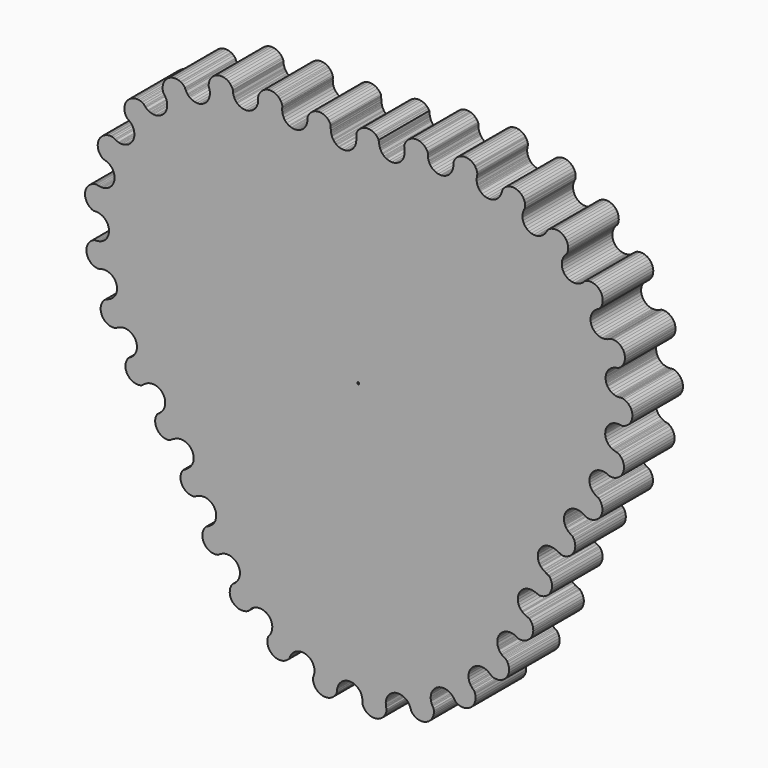
from build123d import *

# Parameters (mm, degrees)
F0_R     = 0.1932686
F1_DEPTH = 12.7


# Not quite as in the source:
# - ends of sketch curves that miss each other by under 0.0002 mm in the source are joined


with BuildPart() as f1:
    # F0 (on Front) → F1 (new body)
    with BuildSketch(Plane.XZ):
        Polygon((-7.2596502, -52.0065254), (-7.258685, -52.006754), (-6.7694048, -52.0724638), (-6.322441, -52.044346), (-6.2991238, -52.0413742), (-6.255639, -52.0358624), (-5.9557158, -51.9563604), (-5.7304432, -51.8810748), (-5.6054752, -51.8198608), (-5.2589684, -51.6220202), (-4.8862488, -51.2983226), (-4.5838364, -50.9081278), (-4.445508, -50.6309884), (-4.3810682, -50.4785376), (-4.38277, -50.2927112), (-4.3556936, -50.1496838), (-4.3439588, -49.9317772), (-4.2878502, -49.7120926), (-4.283329, -49.6734592), (-4.2580052, -49.5952272), (-4.2380408, -49.5170968), (-4.2218102, -49.4535968), (-4.1919906, -49.3912906), (-4.1470072, -49.2522764), (-4.1313354, -49.2039148), (-3.8906704, -48.7730292), (-3.5705796, -48.3973886), (-3.1833566, -48.0913948), (-2.7438604, -47.8668334), (-2.5818084, -47.8209356), (-2.5621996, -47.8124266), (-2.5180036, -47.8028508), (-2.2690074, -47.7323404), (-2.1470366, -47.7225868), (-2.0798282, -47.708058), (-1.9344386, -47.7056196), (-1.8059654, -47.695358), (-1.7770348, -47.6930466), (-1.7760188, -47.693072), (-1.7021048, -47.7017334), (-1.6081248, -47.7001586), (-1.586357, -47.699803), (-1.585341, -47.6998792), (-1.3438886, -47.7437196), (-1.2858496, -47.7505268), (-1.2595606, -47.7590358), (-1.0997692, -47.7880426), (-0.6406896, -47.9692462), (-0.225806, -48.2365558), (0.1289812, -48.5796336), (0.4100068, -48.9853478), (0.6064758, -49.4381028), (0.6447536, -49.614963), (0.6720078, -49.6904772), (0.697357, -49.8581172), (0.7108444, -49.9204742), (0.7113524, -49.9506748), (0.7457948, -50.178462), (0.735965, -50.3910092), (0.7487158, -50.5372878), (0.744474, -50.5759974), (0.7261352, -50.7430532), (0.7559802, -50.8404876), (0.782955, -50.9285748), (0.8832596, -51.1949192), (1.1438382, -51.613816), (1.4810994, -51.9738102), (1.8554192, -52.2419326), (1.8963132, -52.267485), (2.2015704, -52.4057372), (2.3973028, -52.4799306), (2.5652476, -52.5190466), (2.6849324, -52.5390872), (2.931795, -52.5804384), (2.9387546, -52.580667), (2.9445458, -52.5808448), (3.4289492, -52.5660874), (3.4299398, -52.5659604), (3.9106348, -52.4550386), (4.360418, -52.2524736), (4.7620682, -51.9660632), (5.1001168, -51.6067802), (5.361559, -51.1884422), (5.5226712, -50.7633732), (5.5394352, -50.7090426), (5.5643018, -50.5604018), (5.5986172, -50.227865), (5.5079392, -49.938178), (5.489067, -49.762537), (5.4499256, -49.6022376), (5.4286404, -49.1090712), (5.4507638, -48.9657898), (5.4527196, -48.8699302), (5.4956456, -48.675036), (5.5039514, -48.6212642), (5.5129176, -48.5967024), (5.558917, -48.387889), (5.7570878, -47.9358198), (6.0396882, -47.5310962), (6.3957708, -47.189263), (6.8117212, -46.9235028), (7.2715374, -46.7439756), (7.2725026, -46.7436962), (7.7585062, -46.6573362), (8.2520028, -46.6674454), (8.734044, -46.7736174), (8.869172, -46.8328756), (8.9234772, -46.8484966), (9.0284554, -46.9027002), (9.1861386, -46.9718136), (9.2536264, -47.0189306), (9.3620844, -47.0749376), (9.5617284, -47.2340686), (9.5908368, -47.2543886), (9.602597, -47.2666314), (9.7480882, -47.3825824), (10.066655, -47.7596454), (10.1220524, -47.8597976), (10.2047802, -48.009429), (10.20953, -48.0158044), (10.2166674, -48.0309174), (10.3055166, -48.1915724), (10.3282242, -48.2627686), (10.3321104, -48.274859), (10.4206294, -48.4619808), (10.4852216, -48.719613), (10.5323132, -48.8379516), (10.550398, -48.9359956), (10.576814, -48.9758482), (10.8056426, -49.2775748), (11.1644684, -49.5958368), (11.1806228, -49.6084098), (11.452225, -49.7672614), (11.6798852, -49.8815106), (11.7551454, -49.9075202), (12.179046, -50.0242586), (12.6711964, -50.0599202), (13.160883, -49.9989094), (13.6292336, -49.8435122), (13.6301734, -49.8431058), (14.0592048, -49.599342), (14.4324578, -49.2765334), (14.735556, -48.8871514), (14.9568662, -48.4460804), (15.087854, -47.9703384), (15.1098504, -47.6671132), (15.1120094, -47.3911168), (15.0335996, -46.9799924), (14.8506688, -46.710219), (14.7757388, -46.5326476), (14.692884, -46.391068), (14.5313908, -45.9244446), (14.5081244, -45.7555346), (14.4884648, -45.6837034), (14.4779746, -45.536485), (14.4640554, -45.435266), (14.4671034, -45.3838056), (14.4534128, -45.191172), (14.5151094, -44.7012568), (14.6711924, -44.2328046), (14.9156928, -43.8037986), (15.2391872, -43.4307234), (15.6292296, -43.12793), (15.6300932, -43.1273966), (16.071723, -42.9065182), (16.547973, -42.7760384), (17.0405044, -42.7409864), (17.5304196, -42.802683), (17.6652174, -42.8476156), (17.7405538, -42.8621444), (17.88287, -42.9201326), (17.9988718, -42.9587914), (18.051907, -42.9890174), (18.19783, -43.0484788), (18.6099704, -43.3204366), (18.9611508, -43.6675784), (19.0228982, -43.758866), (19.1610488, -43.9143902), (19.3112644, -44.1708032), (19.3882518, -44.2696346), (19.4080384, -44.30903), (19.4484752, -44.34332), (19.7320408, -44.553251), (20.1783696, -44.763817), (20.3202032, -44.7992246), (20.5983078, -44.8686174), (20.6884778, -44.8847972), (20.9026252, -44.8951096), (20.9478372, -44.897294), (21.0921346, -44.894627), (21.2536024, -44.8916044), (21.2793072, -44.887769), (21.2991446, -44.8847972), (21.7514932, -44.7860166), (22.2038164, -44.588684), (22.6089464, -44.3069218), (22.6097338, -44.3062614), (22.9521004, -43.9508646), (23.2185718, -43.535473), (23.3988864, -43.076114), (23.48611, -42.5903898), (23.4769152, -42.0969694), (23.391495, -41.7058348), (23.3520996, -41.5700972), (23.3222546, -41.501695), (23.2649776, -41.391332), (23.1707944, -41.2099252), (22.9620826, -41.0350716), (22.8696266, -40.9200858), (22.7466652, -40.8055318), (22.584029, -40.5798782), (22.5667062, -40.5613362), (22.542373, -40.5220932), (22.4582228, -40.4053294), (22.4253806, -40.3333458), (22.306788, -40.142033), (22.133687, -39.6800832), (22.0540072, -39.1932414), (22.0708474, -38.700202), (22.1835726, -38.2199134), (22.3877886, -37.7708668), (22.675723, -37.3702834), (22.6763834, -37.3695214), (22.7885498, -37.2647464), (22.8252782, -37.2204234), (22.8260148, -37.2197122), (22.9089712, -37.1522752), (23.036911, -37.0327936), (23.1173528, -36.9829588), (23.2088436, -36.9085876), (23.4017058, -36.8066828), (23.4562142, -36.7729008), (23.4886754, -36.7607342), (23.6450124, -36.678108), (24.1177826, -36.5371634), (24.6089424, -36.491164), (25.0996704, -36.5418624), (25.5710436, -36.6873282), (25.7974846, -36.8097562), (25.8438904, -36.8276124), (25.9229098, -36.8775488), (26.0050026, -36.921948), (26.0180328, -36.932743), (26.0432296, -36.9536218), (26.2608822, -37.0912136), (26.390219, -37.214175), (26.4523982, -37.2732808), (26.5811, -37.3673624), (26.6543282, -37.4470422), (26.6817094, -37.4768364), (26.901267, -37.5745756), (27.0568674, -37.6342656), (27.543125, -37.7176538), (28.0362914, -37.7045728), (28.5174436, -37.5955306), (28.895929, -37.4268746), (28.9921188, -37.3777256), (29.1585904, -37.2599712), (29.2089078, -37.2243858), (29.4217852, -37.0561616), (29.4921432, -36.9819682), (29.7636184, -36.6633506), (29.7642026, -36.6625378), (30.0047406, -36.2318046), (30.156658, -35.7624126), (30.214062, -35.2723958), (30.1747682, -34.780601), (30.0403006, -34.3059512), (29.8845478, -34.0011512), (29.7804078, -33.8218272), (29.7726862, -33.8120736), (29.5570402, -33.5674208), (29.3539164, -33.471612), (29.215334, -33.3690722), (29.0514024, -33.2800706), (28.8873946, -33.1436726), (28.8390838, -33.1138276), (28.7354772, -33.017333), (28.6718502, -32.9644248), (28.6509714, -32.9386438), (28.477845, -32.7774046), (28.1891486, -32.3769482), (28.1318208, -32.2513452), (28.1035252, -32.2071238), (28.0550874, -32.083248), (27.9841198, -31.9278508), (27.9686258, -31.8622426), (27.9237186, -31.7473584), (27.8370538, -31.2613802), (27.8468582, -30.7678074), (27.9527762, -30.2856392), (28.1507184, -29.8334176), (28.1512264, -29.8325286), (28.4335982, -29.4276018), (28.7895284, -29.08554), (29.2053772, -28.8195004), (29.6651172, -28.6396684), (29.815282, -28.6128968), (29.8533566, -28.6003746), (29.9557948, -28.5878524), (30.1511208, -28.553029), (30.2282098, -28.554553), (30.3433988, -28.5404814), (30.6410868, -28.5627572), (30.6446936, -28.5628334), (30.6460652, -28.5631382), (30.8356762, -28.5773368), (31.0711088, -28.6427672), (31.090997, -28.645358), (31.1406286, -28.6620966), (31.3113166, -28.7095184), (31.3718956, -28.7401), (31.5587634, -28.8031428), (31.6428882, -28.8515044), (31.7260478, -28.8993072), (31.8625982, -28.953714), (32.0957448, -29.1049202), (32.3817742, -29.16301), (32.6060816, -29.1638736), (32.9381358, -29.1463476), (33.4161892, -29.0247324), (33.8613496, -28.8121852), (34.256472, -28.5168594), (34.586418, -28.1501342), (34.8384622, -27.7261066), (34.8388686, -27.7251922), (35.003359, -27.2601182), (35.0609154, -26.862024), (35.071939, -26.7342874), (35.0595438, -26.4992358), (35.025457, -26.1909814), (35.0120204, -26.1382002), (34.8748604, -25.7047492), (34.6371418, -25.2725174), (34.3196672, -24.8949718), (34.2319864, -24.8247408), (34.0772242, -24.7827546), (33.8386166, -24.6641366), (33.6741516, -24.6085868), (33.4651858, -24.4883686), (33.3699104, -24.449659), (32.9583542, -24.1785902), (32.8722482, -24.0936272), (32.768413, -24.015954), (32.4390004, -23.6494828), (32.1874134, -23.22576), (32.023304, -22.7611178), (31.9529968, -22.273387), (31.9792096, -21.7812874), (32.0145918, -21.6424764), (32.0190622, -21.6029286), (32.0469514, -21.5154764), (32.100901, -21.3037928), (32.1012566, -21.3028276), (32.1419728, -21.2176106), (32.1688206, -21.1334604), (32.169227, -21.132546), (32.2681854, -20.953603), (32.3137784, -20.858226), (32.3412104, -20.8215484), (32.4077076, -20.7013048), (32.725741, -20.3249022), (33.1110844, -20.0177654), (33.548955, -19.7917054), (34.0225126, -19.6554344), (34.5135708, -19.614134), (34.6469716, -19.6292216), (34.759011, -19.6263768), (35.2445828, -19.7102984), (35.3555046, -19.7530212), (35.5625908, -19.8013066), (35.758628, -19.8901558), (35.951414, -19.9469756), (35.9783126, -19.9610726), (36.2037122, -20.0792334), (36.2768134, -20.1053446), (36.7176558, -20.0846944), (37.1956584, -19.9661018), (37.6083322, -19.7720712), (37.6545348, -19.7467982), (37.9135386, -19.5556124), (38.0842266, -19.412839), (38.1856742, -19.3014092), (38.4290316, -18.9990984), (38.6570982, -18.562574), (38.6574792, -18.5616596), (38.7959854, -18.0890418), (38.839648, -17.5984916), (38.7867652, -17.1088304), (38.639369, -16.638905), (38.4031236, -16.2067748), (38.2725422, -16.0506918), (38.1449326, -15.983331), (38.1440944, -15.9826198), (38.0604268, -15.9521906), (37.7552458, -15.7670754), (37.6288554, -15.712313), (37.4094502, -15.5604718), (37.2862094, -15.4979624), (37.1055138, -15.3560272), (37.0331746, -15.3135838), (36.6657636, -14.9869144), (36.6072674, -14.9095968), (36.5503968, -14.8541486), (36.403407, -14.6401282), (36.3691424, -14.59484), (36.3615732, -14.579219), (36.2720636, -14.4488916), (36.07816, -13.9971272), (35.9761028, -13.5162036), (35.9743756, -13.381736), (35.9740708, -13.379831), (35.974274, -13.3735318), (35.969829, -13.024612), (35.9893616, -12.9194052), (35.990403, -12.888468), (36.0133646, -12.7901446), (36.0595926, -12.5412246), (36.0883708, -12.4691648), (36.1022646, -12.4097542), (36.184459, -12.2285252), (36.2419138, -12.0846596), (36.242371, -12.0837706), (36.2680758, -12.0442482), (36.305363, -11.9620284), (36.305871, -11.9611648), (36.4781592, -11.720957), (36.5102902, -11.671554), (36.522914, -11.6586), (36.5924338, -11.5616736), (36.951412, -11.2257586), (37.3690388, -10.9663484), (37.829236, -10.7933998), (38.3143506, -10.7135422), (38.4447034, -10.7178602), (38.4845306, -10.7131866), (38.6149596, -10.7235244), (38.8056882, -10.729849), (38.8627112, -10.743184), (38.9746236, -10.752074), (39.1482326, -10.8011468), (39.1887456, -10.8062522), (39.3150852, -10.8483146), (39.4476986, -10.885805), (39.4852906, -10.9050074), (39.6551912, -10.9615732), (39.734617, -11.0068106), (39.9984722, -11.1129826), (40.0716242, -11.1607854), (40.4145496, -11.3236248), (40.455088, -11.3537746), (40.4686262, -11.3580672), (40.7699972, -11.5241324), (40.7989024, -11.5286536), (40.9657042, -11.5443762), (41.1111954, -11.5382802), (41.5002726, -11.4983006), (41.9706298, -11.3534698), (42.4036998, -11.1196374), (42.7828456, -10.8058204), (43.0934622, -10.4240584), (43.094021, -10.4232202), (43.3241958, -9.9881944), (43.4650896, -9.5166434), (43.5112668, -9.0266266), (43.4609748, -8.5370416), (43.3381404, -8.1380838), (43.3004468, -8.0376268), (43.2036728, -7.8583536), (43.0190402, -7.5606656), (42.9690784, -7.5071986), (42.8991014, -7.4709274), (42.7899068, -7.3836022), (42.5343066, -7.2323706), (42.4269408, -7.1361808), (42.2521888, -7.0189344), (42.128821, -6.895084), (42.0530274, -6.8376546), (41.7257484, -6.4690244), (41.6322764, -6.30936), (41.6313112, -6.3081408), (41.6296348, -6.3048642), (41.476676, -6.0436252), (41.4348676, -5.9228228), (41.4191196, -5.8919618), (41.4074102, -5.8689748), (41.3684974, -5.7311544), (41.3154114, -5.5778146), (41.3060388, -5.5099458), (41.273476, -5.394579), (41.2510986, -5.1113436), (41.2481014, -5.0894742), (41.2486348, -5.0802032), (41.2346648, -4.9031652), (41.2924752, -4.4136056), (41.4446974, -3.944747), (41.6854386, -3.514598), (41.6859974, -3.5137852), (42.0060628, -3.1388558), (42.393108, -2.8335732), (42.8322486, -2.6096722), (43.3066698, -2.475738), (43.7980836, -2.4369268), (43.9709052, -2.457323), (44.0109864, -2.4565356), (44.1029598, -2.4729186), (44.2876178, -2.4947372), (44.3635384, -2.5193752), (44.4963042, -2.543048), (44.9553838, -2.7225752), (45.0508116, -2.7836114), (45.2269606, -2.8648914), (45.3893174, -2.9828998), (45.5681842, -3.0788356), (45.5994262, -3.1045658), (45.7162408, -3.2007048), (45.8099414, -3.2335724), (45.9838552, -3.283712), (46.0102712, -3.2874458), (46.0259938, -3.289681), (46.4874864, -3.32867), (46.9778842, -3.2735012), (47.448089, -3.123692), (47.8800414, -2.885059), (48.2571552, -2.5667208), (48.5649016, -2.1809456), (48.565435, -2.180082), (48.792003, -1.741678), (48.9085382, -1.337437), (48.9311442, -1.2384786), (48.9555282, -0.9500108), (48.962437, -0.7062216), (48.946054, -0.5606796), (48.881411, -0.1797304), (48.8792266, -0.1728216), (48.7052112, 0.2834132), (48.442753, 0.7013448), (48.2199442, 0.9371076), (48.1291138, 1.0231628), (47.7640904, 1.1932412), (47.6645732, 1.2661646), (47.5241874, 1.3407898), (47.3851986, 1.4543278), (47.3601796, 1.46939), (47.302293, 1.5220696), (47.1420698, 1.6529558), (47.0929716, 1.7125188), (46.9952324, 1.8014696), (46.7020656, 2.1983446), (46.4919822, 2.644775), (46.3730086, 3.1236412), (46.3497676, 3.6165028), (46.4230974, 4.1044368), (46.5902294, 4.5686726), (46.5906612, 4.569587), (46.6630258, 4.6897798), (46.670595, 4.707763), (46.671103, 4.708652), (46.7003892, 4.7518828), (46.8451438, 4.9923192), (46.9167972, 5.0710592), (46.947963, 5.1170586), (47.0522554, 5.2199286), (47.177198, 5.3572664), (47.23384, 5.3991002), (47.2992196, 5.4635908), (47.5013782, 5.5967122), (47.574073, 5.6504078), (47.6050864, 5.6650128), (47.7113092, 5.734939), (48.1684076, 5.9206892), (48.6529888, 6.0136786), (49.1463838, 6.0103766), (49.3316514, 5.9722004), (49.3743742, 5.9695842), (49.4815876, 5.9413394), (49.6296442, 5.9108594), (49.683416, 5.8881518), (49.8514878, 5.8438796), (50.0254524, 5.7589674), (50.1444006, 5.7204864), (50.3696986, 5.5946802), (50.418238, 5.587492), (50.8447802, 5.5471314), (51.3109718, 5.5948326), (51.3251704, 5.5972964), (51.349148, 5.6014366), (51.4005068, 5.6172354), (51.6494522, 5.6937656), (51.8309352, 5.7636918), (51.8877296, 5.7855612), (51.9729212, 5.8315098), (52.337081, 6.061837), (52.6948908, 6.4021208), (52.9794216, 6.805676), (53.1797514, 7.2569832), (53.1800562, 7.2579484), (53.2885142, 7.7396594), (53.300884, 8.2332576), (53.2167338, 8.71982), (53.039264, 9.1806014), (52.7753326, 9.597898), (52.436522, 9.954133), (52.4340836, 9.9563428), (52.2602968, 10.0788978), (51.9669776, 10.257028), (51.8575036, 10.2684834), (51.746277, 10.303002), (51.4732016, 10.3498904), (51.2649724, 10.4297988), (51.2055364, 10.444099), (51.0965958, 10.494391), (51.012598, 10.526649), (50.9737868, 10.5511092), (50.7576074, 10.6509312), (50.3586496, 10.941177), (50.0239792, 11.3036858), (49.766474, 11.724513), (49.5959892, 12.1874788), (49.5191288, 12.6748286), (49.5262408, 12.8531874), (49.5243358, 12.8745742), (49.5287554, 12.9157984), (49.5339116, 13.0449828), (49.5388138, 13.1677918), (49.5389408, 13.1687824), (49.5693954, 13.2952998), (49.5768884, 13.3651244), (49.5770916, 13.366115), (49.6177824, 13.4962138), (49.6544092, 13.6484614), (49.688369, 13.721969), (49.7243354, 13.8369802), (49.8359684, 14.0416026), (49.8612668, 14.096365), (49.8795802, 14.1215618), (49.9606062, 14.2700756), (50.2768616, 14.6487642), (50.6608842, 14.9584918), (51.0979674, 15.1873204), (51.5712964, 15.326487), (51.8522966, 15.35176), (51.868832, 15.3554176), (51.9010138, 15.3561288), (52.0626848, 15.3706576), (52.1475208, 15.3615644), (52.2588236, 15.3640282), (52.3620746, 15.3663142), (52.6918936, 15.3082244), (52.784121, 15.3039572), (52.8367244, 15.290927), (53.0942042, 15.3414984), (53.3496012, 15.4093164), (53.7929328, 15.6266896), (54.1853374, 15.9263842), (54.5117274, 16.2968686), (54.7595552, 16.7239188), (54.9193466, 17.191101), (54.9822624, 17.6608232), (54.9843198, 17.6910746), (54.9611296, 18.0572918), (54.9387776, 18.2306214), (54.8823134, 18.4432194), (54.7798244, 18.74774), (54.7469314, 18.8148214), (54.5260784, 19.199606), (54.2014918, 19.5716652), (53.810535, 19.8732648), (53.3682702, 20.0927716), (53.0698456, 20.1735436), (52.8845272, 20.2110594), (52.7396456, 20.1792586), (52.6731738, 20.1779378), (52.6083022, 20.1766678), (52.3687548, 20.1398124), (52.1527278, 20.1492612), (52.0955016, 20.1441558), (51.9768328, 20.1569574), (51.8757408, 20.161377), (51.828446, 20.1729594), (51.6048498, 20.197064), (51.1339592, 20.3446888), (50.70094, 20.5813406), (50.3223784, 20.8979262), (50.012854, 21.2822536), (49.9418102, 21.418169), (49.9192042, 21.4502492), (49.886362, 21.5243156), (49.7842794, 21.7196162), (49.7542312, 21.8220544), (49.7190522, 21.9013278), (49.6798092, 22.0758258), (49.6453922, 22.1931484), (49.6452144, 22.194139), (49.639982, 22.2528638), (49.6107466, 22.3827848), (49.6106196, 22.3837754), (49.6037616, 22.6589844), (49.601374, 22.6856798), (49.602771, 22.698583), (49.598326, 22.8770942), (49.6825016, 23.3633518), (49.859946, 23.8238284), (50.1238012, 24.240871), (50.4639326, 24.5984014), (50.8672846, 24.8827036), (51.050698, 24.9640852), (51.1080004, 24.999188), (51.2371086, 25.046813), (51.3183632, 25.0828556), (51.360705, 25.0923806), (51.5709916, 25.1699268), (51.8110724, 25.2079252), (51.9375644, 25.2454664), (52.1076936, 25.261189), (52.3086076, 25.3728728), (52.5398492, 25.5213612), (52.895246, 25.8639818), (53.1769574, 26.2693658), (53.3741884, 26.721943), (53.4723594, 27.172412), (53.4795984, 27.2198084), (53.4859484, 27.5664676), (53.4772362, 27.7595076), (53.4419302, 27.9557988), (53.3603454, 28.2871418), (53.3408382, 28.3367734), (53.1467568, 28.75153), (52.8543012, 29.1492432), (52.4898874, 29.4822372), (52.0674854, 29.7377612), (51.6033512, 29.9059854), (51.115341, 29.9804074), (50.8974852, 29.9705776), (50.60823, 29.9391832), (50.3679968, 29.8025312), (50.3038364, 29.7811952), (50.2108216, 29.7502834), (50.0548656, 29.6741088), (49.5776504, 29.548201), (49.5631724, 29.547312), (49.4514632, 29.5404286), (49.337214, 29.517848), (49.0907578, 29.5181782), (49.0850428, 29.5178226), (49.0823758, 29.5181782), (48.8436666, 29.5185084), (48.3597458, 29.6154094), (47.904019, 29.8048934), (47.4940122, 30.0796198), (47.1454988, 30.429073), (46.8718392, 30.839791), (46.8713566, 30.84068), (46.6830918, 31.2968894), (46.5874608, 31.7810642), (46.587664, 31.9407286), (46.5827364, 31.9778634), (46.5878164, 32.0569336), (46.5880958, 32.2746116), (46.6083142, 32.3755512), (46.6144356, 32.4703948), (46.6662008, 32.6645016), (46.6850222, 32.7585324), (46.7024466, 32.800417), (46.741588, 32.9472544), (46.9593676, 33.3901542), (47.2593416, 33.7820508), (47.457741, 33.9564726), (47.471076, 33.9717888), (47.5049342, 33.9979508), (47.6300292, 34.1079074), (47.698279, 34.1474298), (47.807499, 34.2318594), (47.8615248, 34.2736424), (48.0947222, 34.389695), (48.1974906, 34.4592402), (48.301529, 34.5030552), (48.3490524, 34.552509), (48.5673908, 34.8103444), (48.5944672, 34.8423484), (48.8207304, 35.2503994), (48.8375452, 35.285807), (48.9274866, 35.5667056), (48.9656882, 35.7182674), (48.9940854, 35.8308656), (48.9978954, 35.8643682), (49.001045, 35.8919526), (49.0238796, 36.3427772), (48.9522262, 36.8308636), (48.7867198, 37.295582), (48.5337358, 37.7190762), (48.5331516, 37.719889), (48.2023928, 38.085903), (47.80661, 38.3803652), (47.360967, 38.5919472), (46.8826342, 38.712521), (46.3912458, 38.7373876), (46.3893408, 38.7373622), (46.238541, 38.7152388), (46.1154272, 38.697154), (45.8173074, 38.6339842), (45.4502012, 38.4765296), (45.4361296, 38.4596386), (45.3374252, 38.380035), (45.1353682, 38.16731), (44.9689982, 38.049835), (44.8868292, 37.9736858), (44.466256, 37.7152916), (44.2689488, 37.6422158), (44.2631322, 37.6391424), (44.2500258, 37.6352054), (44.0033664, 37.5438924), (43.8788048, 37.5240042), (43.7902858, 37.4974866), (43.7647588, 37.4950736), (43.5985158, 37.4792748), (43.5159404, 37.4660922), (43.4758338, 37.4676162), (43.2988974, 37.4508014), (42.8078392, 37.5008902), (42.3359834, 37.6457972), (41.9014656, 37.8799852), (41.5209736, 38.1944626), (41.5202624, 38.1951738), (41.208452, 38.5777994), (40.9772612, 39.0139428), (40.8356054, 39.4867892), (40.7889456, 39.9781776), (40.839009, 40.4692358), (40.8770328, 40.59301), (40.8926284, 40.6866598), (40.962961, 40.872791), (40.9839414, 40.9410916), (41.0001212, 40.9711144), (41.067101, 41.1484064), (41.32834, 41.567227), (41.4170622, 41.6616896), (41.527349, 41.815893), (41.750361, 42.0251382), (41.820973, 42.1117522), (41.8232844, 42.1136572), (41.9823646, 42.4755056), (42.044874, 42.7579536), (42.082974, 43.0038256), (42.089324, 43.0447704), (42.0683182, 43.5377844), (41.951529, 44.0172348), (41.7434522, 44.4646812), (41.4520888, 44.8629532), (41.0886148, 45.1967092), (41.0878274, 45.1973188), (40.6662128, 45.4537572), (40.2026882, 45.6230228), (39.715059, 45.6985878), (39.2865864, 45.6803252), (39.2449304, 45.6758548), (39.1913618, 45.6701144), (39.0367266, 45.6324462), (38.9626856, 45.6144122), (38.6432298, 45.5144378), (38.210109, 45.2779892), (37.934773, 45.0479668), (37.9234446, 45.0371718), (37.9090682, 45.0032882), (37.8258578, 44.8810634), (37.6919236, 44.6161414), (37.6106944, 44.5124078), (37.551741, 44.4371222), (37.5007632, 44.3509654), (37.1712744, 43.983148), (36.7763806, 43.6867046), (36.7411508, 43.6697882), (36.6249204, 43.6140098), (36.580445, 43.5849776), (36.4824518, 43.5456076), (36.3312456, 43.4730144), (36.2495338, 43.452034), (36.1222544, 43.4009038), (35.8542336, 43.350561), (35.8529636, 43.3502562), (35.8523286, 43.3502054), (35.636962, 43.3097686), (35.143186, 43.3150518), (34.659951, 43.4165756), (34.2058244, 43.610403), (34.2049354, 43.610911), (33.7973162, 43.8896252), (33.451927, 44.2425074), (33.1820012, 44.655994), (32.9979274, 45.1141846), (32.9067922, 45.599477), (32.908748, 45.7802742), (32.9013566, 45.8412342), (32.9107038, 45.964221), (32.9121008, 46.093253), (32.9252834, 46.1560926), (32.9387962, 46.3335878), (33.071562, 46.8092028), (33.1392784, 46.9429592), (33.2036928, 47.1268552), (33.372933, 47.413545), (33.384363, 47.440469), (33.4362044, 47.8362772), (33.4115918, 48.2081332), (33.4009746, 48.2877368), (33.3874872, 48.388778), (33.3619856, 48.483647), (33.2733904, 48.7430826), (33.2235556, 48.889031), (32.9760072, 49.3159542), (32.6499474, 49.6863878), (32.257873, 49.9860824), (31.8148716, 50.2035318), (31.8139318, 50.2038874), (31.3370214, 50.3307096), (30.8445154, 50.3620786), (30.3553622, 50.2967752), (29.8883578, 50.1372886), (29.5571418, 49.9452392), (29.4181022, 49.8516148), (29.328491, 49.7727224), (29.324808, 49.7694712), (29.0349178, 49.4774728), (29.010356, 49.4404142), (28.8532062, 49.203356), (28.842589, 49.127283), (28.8149792, 49.0479334), (28.7976818, 48.9981748), (28.7538922, 48.7724196), (28.688157, 48.611536), (28.6601662, 48.4991156), (28.4498542, 48.052863), (28.3459174, 47.9123248), (28.297886, 47.826422), (28.1810968, 47.6894398), (28.156535, 47.6562166), (28.1397964, 47.6410274), (27.9777952, 47.4510354), (27.590623, 47.145321), (27.1512284, 46.921039), (26.6765278, 46.7867492), (26.1847584, 46.7476586), (25.6948178, 46.8052658), (25.6938272, 46.8054944), (25.2245368, 46.9575896), (24.7939306, 47.19828), (24.4185694, 47.5183962), (24.3033296, 47.6643446), (24.2816888, 47.6855028), (24.2733322, 47.6936816), (24.229314, 47.7580706), (24.1301778, 47.8836228), (24.112855, 47.9055684), (24.0669318, 47.9955606), (23.994872, 48.1008944), (23.9017302, 48.3191312), (23.8885476, 48.3449376), (23.8843058, 48.3599236), (23.8195866, 48.5115616), (23.8012224, 48.5546146), (23.6997748, 49.0374178), (23.6944916, 49.5307112), (23.7113572, 49.6204748), (23.7161832, 49.7047774), (23.7254034, 49.8660674), (23.8006128, 50.1563894), (23.8195866, 50.3081544), (23.8383064, 50.3644662), (23.8302546, 50.4569222), (23.8074454, 50.6191774), (23.795101, 50.707163), (23.6324902, 51.1729482), (23.4578398, 51.4694932), (23.4181904, 51.529361), (23.3453178, 51.6393176), (23.2997756, 51.6903462), (23.2715816, 51.7219184), (22.9811834, 52.0145772), (22.5720148, 52.290218), (22.1169484, 52.4807688), (21.633434, 52.5788636), (21.632418, 52.5789652), (21.1390738, 52.5808448), (20.6548482, 52.486433), (20.198334, 52.2993874), (20.02028, 52.1814044), (19.7975982, 52.0338304), (19.7837044, 52.023518), (19.5831206, 51.8244582), (19.3936366, 51.6151622), (19.3838322, 51.6005826), (19.1370458, 51.1882644), (19.0486284, 50.9407414), (19.0465456, 50.9336802), (19.0481458, 50.920396), (19.035141, 50.7495302), (19.0508128, 50.502566), (19.0286386, 50.3367802), (19.0241936, 50.3035824), (19.0250826, 50.1762014), (18.9321186, 49.6913662), (18.8919358, 49.5924078), (18.8590936, 49.4612168), (18.6480958, 49.0149134), (18.3540908, 48.6183432), (17.9883816, 48.2867716), (17.8467512, 48.2018594), (17.8399186, 48.1962968), (17.8200304, 48.185832), (17.564989, 48.0328986), (17.4551848, 47.9935794), (17.4031656, 47.9661728), (17.2594524, 47.9235262), (17.1002198, 47.8665032), (17.0345862, 47.8567496), (16.9299382, 47.8256854), (16.6526972, 47.8000314), (16.6119048, 47.7939862), (16.6108888, 47.7939354), (16.5950392, 47.7947228), (16.438372, 47.7802194), (16.437356, 47.7802194), (15.946374, 47.8315274), (15.474823, 47.9776282), (15.0408386, 48.2129338), (14.6611086, 48.528351), (14.3501872, 48.9118148), (14.264894, 49.0737398), (14.2450312, 49.1011464), (14.208506, 49.18075), (14.1200632, 49.3485678), (14.0992352, 49.4187988), (14.039088, 49.5497866), (13.9246356, 50.029999), (13.9209272, 50.128297), (13.886434, 50.3179334), (13.8900408, 50.5368814), (13.8716004, 50.6818646), (13.8846814, 50.8686562), (13.8443462, 50.9972564), (13.7930636, 51.1332734), (13.5323834, 51.5520686), (13.1949952, 51.9119358), (12.7938784, 52.1990574), (12.4426472, 52.3580106), (12.3012962, 52.4124682), (12.2381518, 52.4271748), (12.0978422, 52.4598138), (11.7653054, 52.5173956), (11.740769, 52.518183), (11.2650778, 52.506372), (11.2640872, 52.506245), (10.782808, 52.3980156), (10.3319072, 52.1979652), (9.9286822, 51.91379), (9.5886524, 51.556412), (9.3248988, 51.1395726), (9.2633546, 50.9799082), (9.2131388, 50.8496316), (9.1389454, 50.6180598), (9.1375992, 50.6062996), (9.158351, 50.403633), (9.2015564, 50.2251218), (9.2123514, 49.9627652), (9.237853, 49.8201188), (9.2358972, 49.720627), (9.2328492, 49.5644678), (9.239377, 49.508918), (9.2293186, 49.3829594), (9.2282264, 49.327435), (9.2229686, 49.303432), (9.2001594, 49.0177074), (9.146667, 48.8287822), (9.1432634, 48.804576), (9.1248484, 48.7517948), (9.065895, 48.543591), (9.022842, 48.4593392), (8.9809828, 48.3392988), (8.7310214, 47.9146108), (8.4030312, 47.5468442), (8.0095852, 47.2501468), (7.5658218, 47.0358978), (7.0887844, 46.9123268), (7.0877938, 46.9121744), (6.5958212, 46.8840566), (6.1078364, 46.9524588), (5.6425338, 47.1147648), (5.520309, 47.1866976), (5.469636, 47.207805), (5.3638704, 47.2787726), (5.2178458, 47.3647008), (5.1633628, 47.413291), (5.060442, 47.4823536), (4.8574706, 47.6861124), (4.8500792, 47.692691), (4.8475138, 47.6960946), (4.7373794, 47.8066862), (4.7126652, 47.8314766), (4.4396914, 48.2417374), (4.3608498, 48.433101), (4.3264074, 48.4920544), (4.2739056, 48.6441496), (4.2519854, 48.6973626), (4.247261, 48.7213402), (4.1656254, 48.957865), (4.146804, 49.0953806), (4.1096946, 49.2271558), (4.0866314, 49.3089184), (4.0690292, 49.5336322), (4.0217344, 49.7475764), (4.0171116, 49.96561), (3.8306502, 50.270156), (3.7937694, 50.3229118), (3.6323016, 50.4977146), (3.5273234, 50.5984002), (3.3960054, 50.7243334), (2.9808678, 50.9893062), (2.5219914, 51.1681984), (2.0370546, 51.254152), (1.5446756, 51.2438142), (1.5436596, 51.2437126), (1.0627614, 51.1375406), (0.6118098, 50.939573), (0.2081276, 50.6574298), (-0.1327404, 50.3019568), (-0.3119628, 50.0212106), (-0.4238752, 49.8197632), (-0.4507484, 49.7508276), (-0.4810506, 49.656492), (-0.476123, 49.3723168), (-0.4570476, 49.24933), (-0.470154, 48.940593), (-0.4555744, 48.7852466), (-0.4799584, 48.5484678), (-0.4754626, 48.4119174), (-0.5119116, 48.1908866), (-0.513588, 48.1320348), (-0.542544, 48.0051618), (-0.5554726, 47.9268536), (-0.5680964, 47.8932494), (-0.6230112, 47.6527368), (-0.6783578, 47.5290642), (-0.683387, 47.5109286), (-0.7110476, 47.4560646), (-0.823849, 47.203995), (-0.8727948, 47.135034), (-0.904621, 47.0718896), (-1.0468102, 46.8898478), (-1.1083798, 46.8030814), (-1.1320526, 46.780704), (-1.2072366, 46.684438), (-1.5796514, 46.3634582), (-2.0075144, 46.12132), (-2.4743918, 45.9672944), (-2.9623512, 45.907325), (-2.9633672, 45.9072996), (-3.453638, 45.9436724), (-3.9274242, 46.0749904), (-4.050157, 46.1368394), (-4.0570912, 46.1391), (-4.0778176, 46.150784), (-4.3664632, 46.2962244), (-4.444619, 46.3572606), (-4.485513, 46.380273), (-4.6016164, 46.4798664), (-4.7539148, 46.59884), (-4.792599, 46.6437472), (-4.858639, 46.7003892), (-5.033645, 46.9234266), (-5.0432208, 46.934501), (-5.0748692, 46.9712548), (-5.0844196, 46.988095), (-5.1621436, 47.087155), (-5.3843682, 47.525686), (-5.41528, 47.6362014), (-5.4474618, 47.7077024), (-5.497703, 47.9254566), (-5.5052468, 47.9445066), (-5.5123588, 47.9833432), (-5.5167784, 47.9991674), (-5.5177944, 48.0125532), (-5.5579772, 48.1867464), (-5.5596536, 48.2421184), (-5.5936642, 48.4281226), (-5.5922926, 48.5168956), (-5.6302656, 48.8321858), (-5.6254396, 48.8952286), (-5.6417718, 49.1705392), (-5.651119, 49.3279938), (-5.6442102, 49.3781588), (-5.6526684, 49.4209832), (-5.6525668, 49.556543), (-5.7333896, 49.7431822), (-6.0132976, 50.1480074), (-6.3667894, 50.4904502), (-6.7803268, 50.757328), (-7.2379586, 50.9384046), (-7.7221334, 51.0267458), (-7.7231494, 51.026822), (-8.215249, 51.0189988), (-8.6317582, 50.9292098), (-8.7232744, 50.9036574), (-8.9177622, 50.819431), (-8.9945464, 50.7861824), (-9.2091002, 50.6774958), (-9.33196, 50.5925582), (-9.6357948, 50.3541792), (-9.64057, 50.3492516), (-9.9579938, 49.9793768), (-10.1994716, 49.5505232), (-10.211435, 49.5140234), (-10.2510844, 49.392967), (-10.2466394, 49.2240824), (-10.2670356, 49.105312), (-10.275697, 48.8171236), (-10.3056182, 48.6871518), (-10.3223314, 48.4956358), (-10.3713026, 48.327564), (-10.3806752, 48.263175), (-10.4327706, 48.1164392), (-10.4601772, 48.0223576), (-10.4790748, 47.9860356), (-10.5456228, 47.7986344), (-10.7979972, 47.375191), (-11.1281464, 47.0091516), (-11.5233704, 46.7145116), (-11.9684546, 46.5026756), (-12.0583198, 46.4799426), (-12.112498, 46.4662266), (-12.132818, 46.4579716), (-12.1834402, 46.4482688), (-12.4463302, 46.3817208), (-12.5614938, 46.3757772), (-12.616942, 46.36516), (-12.7497586, 46.3660744), (-12.938633, 46.3563208), (-12.939649, 46.3563716), (-13.0189224, 46.3679286), (-13.1098798, 46.3685636), (-13.1108704, 46.3686652), (-13.3211062, 46.4119976), (-13.4274306, 46.427517), (-13.4704836, 46.4427824), (-13.5936736, 46.4681824), (-13.8662664, 46.5833206), (-13.8919712, 46.5924392), (-13.901928, 46.5983828), (-14.0477748, 46.6599778), (-14.4557496, 46.9366854), (-14.8019008, 47.2876626), (-15.0729188, 47.699422), (-15.2583896, 48.1561394), (-15.2933908, 48.3386638), (-15.3122884, 48.3944168), (-15.3299922, 48.5295702), (-15.3512012, 48.6402634), (-15.350871, 48.6889552), (-15.3763218, 48.883189), (-15.3655776, 49.0457236), (-15.378049, 49.222406), (-15.3489914, 49.4522506), (-15.3510996, 49.657254), (-15.3449528, 49.6898168), (-15.4022552, 49.9418102), (-15.6034486, 50.3924316), (-15.8623762, 50.7580392), (-15.9019748, 50.807747), (-16.1445956, 51.0375154), (-16.2950906, 51.1647694), (-16.4633402, 51.2706874), (-16.7541194, 51.4316472), (-16.8007792, 51.4495034), (-16.815181, 51.4549898), (-17.2407326, 51.5909306), (-17.7310796, 51.6465058), (-17.7320956, 51.6465312), (-18.223865, 51.6053578), (-18.6981846, 51.469036), (-19.1367664, 51.2428236), (-19.5227956, 50.935382), (-19.8414132, 50.5585476), (-20.0804018, 50.126773), (-20.1547476, 49.8940836), (-20.2197208, 49.6434364), (-20.2003152, 49.4854484), (-20.206081, 49.407826), (-20.1885296, 49.1570772), (-20.2044046, 49.03216), (-20.2021948, 48.9011214), (-20.2902058, 48.4156258), (-20.3343764, 48.303688), (-20.3490576, 48.2417374), (-20.419568, 48.087661), (-20.471257, 47.9566224), (-20.4999082, 47.912147), (-20.5543912, 47.7930972), (-20.8433162, 47.3931234), (-21.2047328, 47.0572084), (-21.6247218, 46.79823), (-22.0871542, 46.6261958), (-22.5742754, 46.547659), (-22.5752914, 46.5476082), (-23.0683562, 46.5656168), (-23.548467, 46.679485), (-23.9971072, 46.8848186), (-24.397081, 47.1737436), (-24.5057422, 47.2906344), (-24.5207536, 47.3027756), (-24.5531132, 47.3416122), (-24.732996, 47.5351602), (-24.7859804, 47.621063), (-24.8366026, 47.6818198), (-24.9355102, 47.8635822), (-24.9919744, 47.9551492), (-25.0063, 47.9936556), (-25.0360688, 48.0483418), (-25.0724416, 48.11522), (-25.2192282, 48.5863138), (-25.232233, 48.7089704), (-25.2660404, 48.8429554), (-25.2790452, 49.0988604), (-25.2967744, 49.1902496), (-25.2962664, 49.2984028), (-25.4223266, 49.587277), (-25.5250442, 49.7925852), (-25.8278376, 50.1826022), (-26.2009128, 50.5060712), (-26.6299188, 50.7505208), (-27.098371, 50.9066038), (-27.5882608, 50.968275), (-28.0807922, 50.9331976), (-28.0817828, 50.9330198), (-28.5580074, 50.8025146), (-28.9996118, 50.5816362), (-29.3537386, 50.3067066), (-29.4057578, 50.26025), (-29.609034, 50.0257826), (-29.7556682, 49.8310154), (-29.8227242, 49.7133626), (-29.9987716, 49.3480344), (-30.122241, 48.8699556), (-30.1488602, 48.3981506), (-30.1484792, 48.3658164), (-30.146752, 48.3534466), (-30.1384208, 48.3140004), (-30.0362112, 48.0628452), (-30.0068488, 47.9102928), (-29.9491146, 47.7363282), (-29.8880276, 47.2467686), (-29.9005752, 47.0728548), (-29.8973748, 47.017305), (-29.9123608, 46.90999), (-29.9235876, 46.7546944), (-29.944822, 46.67758), (-29.9655992, 46.5286852), (-30.1278544, 46.0627476), (-30.3778666, 45.6374246), (-30.70606, 45.2690484), (-31.0998108, 44.9717922), (-31.5439806, 44.7570352), (-31.5449204, 44.756705), (-32.0224658, 44.6327276), (-32.5149972, 44.6043304), (-33.003617, 44.6725548), (-33.4695546, 44.8347846), (-33.8948776, 45.0847968), (-34.0430866, 45.2168514), (-34.0778592, 45.240575), (-34.1343742, 45.2981822), (-34.2632538, 45.4129902), (-34.3174828, 45.4848214), (-34.42335, 45.592746), (-34.6935044, 46.0055722), (-34.7798644, 46.2198212), (-34.8447106, 46.3353658), (-34.918269, 46.5610448), (-34.9312992, 46.5855558), (-34.936684, 46.594268), (-35.2733864, 46.9553798), (-35.565461, 47.1656918), (-35.7350568, 47.271686), (-35.7874824, 47.2955874), (-35.8458262, 47.3221812), (-36.2313474, 47.468282), (-36.7183162, 47.5498414), (-37.2118382, 47.53483), (-37.6929396, 47.4238066), (-38.1431546, 47.2210638), (-38.1440182, 47.2205558), (-38.546024, 46.9338914), (-38.8843774, 46.5742782), (-39.1460736, 46.1555846), (-39.3210796, 45.6938888), (-39.4026136, 45.20692), (-39.3926568, 44.879514), (-39.3690856, 44.6331848), (-39.360475, 44.5958722), (-39.2284712, 44.1562744), (-39.0142222, 43.906059), (-38.9328406, 43.7612028), (-38.8382002, 43.635295), (-38.6243576, 43.190541), (-38.5833874, 43.0313592), (-38.5604512, 42.9746156), (-38.5367784, 42.850181), (-38.5013708, 42.71264), (-38.4975608, 42.6441362), (-38.4682238, 42.4898312), (-38.4723386, 41.99636), (-38.5726686, 41.5131758), (-38.7653022, 41.0588714), (-39.0428988, 40.6508458), (-39.394765, 40.304847), (-39.3955524, 40.304212), (-39.8081246, 40.0334734), (-40.265604, 39.8484598), (-40.7504138, 39.7562324), (-41.2438596, 39.7603726), (-41.4407096, 39.8012412), (-41.457118, 39.8024096), (-41.4897316, 39.8114012), (-41.7270438, 39.8606772), (-41.8356288, 39.9067274), (-41.9328854, 39.9335244), (-42.1181784, 40.0265392), (-42.1813736, 40.0533362), (-42.2089834, 40.0721068), (-42.2641014, 40.0997928), (-42.3739056, 40.1549108), (-42.7632622, 40.4580852), (-42.8634652, 40.5739854), (-42.9889666, 40.6854152), (-43.2017424, 40.9662884), (-43.2072796, 40.9718764), (-43.4813456, 41.1244542), (-43.628183, 41.2061914), (-43.919521, 41.3000444), (-44.1870846, 41.3678624), (-44.2037216, 41.3697928), (-44.6853564, 41.3948118), (-45.1738746, 41.3237426), (-45.6391518, 41.1587188), (-46.063281, 40.9061158), (-46.4300062, 40.5756364), (-46.4306666, 40.5748744), (-46.7258654, 40.1791932), (-46.938184, 39.7335248), (-47.059469, 39.2549888), (-47.0850722, 38.7619748), (-47.0335356, 38.4077464), (-46.9924384, 38.2125982), (-46.9504522, 38.0942596), (-46.789975, 37.7188984), (-46.5539074, 37.3740934), (-46.5385404, 37.3544338), (-46.4556094, 37.3093234), (-46.3563462, 37.226621), (-46.1368648, 37.0886482), (-45.9871826, 36.9470686), (-45.9189582, 36.8979196), (-45.7976224, 36.76777), (-45.7783184, 36.7495074), (-45.7710286, 36.7392204), (-45.5824336, 36.5369094), (-45.3228202, 36.1171744), (-45.2578724, 35.9433622), (-45.2511668, 35.93084), (-45.2424546, 35.9021126), (-45.1500748, 35.6548436), (-45.1300342, 35.5316536), (-45.1078346, 35.4585778), (-45.091985, 35.2978212), (-45.0708268, 35.1677224), (-45.0730112, 35.1054416), (-45.0593968, 34.967418), (-45.0880988, 34.6756228), (-45.0881496, 34.6744798), (-45.0882766, 34.6739718), (-45.107733, 34.4762582), (-45.2509128, 34.0039452), (-45.483526, 33.5686654), (-45.4840848, 33.5678272), (-45.7971398, 33.1862684), (-46.178597, 32.8731372), (-46.613826, 32.6404224), (-47.0860882, 32.4970902), (-47.577248, 32.4486524), (-47.7939862, 32.469963), (-47.81296, 32.4693026), (-47.8525586, 32.4757288), (-48.0684078, 32.4969632), (-48.1666804, 32.5267574), (-48.300132, 32.5484236), (-48.7624628, 32.7210928), (-48.9099098, 32.812228), (-49.0572552, 32.8781156), (-49.2988346, 33.0494386), (-49.6234974, 33.1187298), (-49.7961158, 33.144333), (-49.8021356, 33.1444346), (-49.8186456, 33.1446378), (-50.2960132, 33.1212444), (-50.7745238, 33.0014072), (-51.220497, 32.7905364), (-51.6167624, 32.4966838), (-51.9480546, 32.1312032), (-52.201699, 31.70809), (-52.2021308, 31.7071756), (-52.3446248, 31.309056), (-52.3732506, 31.2097166), (-52.4145764, 30.9312818), (-52.436649, 30.6703222), (-52.4353028, 30.6428648), (-52.4306292, 30.5477164), (-52.384833, 30.1406306), (-52.2351254, 29.6706036), (-51.9965686, 29.2388036), (-51.6783574, 28.8618422), (-51.4800342, 28.7036002), (-51.3148834, 28.5881318), (-51.095656, 28.5427928), (-50.9382268, 28.4761686), (-50.7485904, 28.424124), (-50.524029, 28.3116782), (-50.5116846, 28.307411), (-50.4882658, 28.2937458), (-50.30724, 28.2031186), (-50.2303796, 28.1434032), (-50.0852694, 28.0587958), (-49.715547, 27.7317454), (-49.4167414, 27.3388582), (-49.200308, 26.8952218), (-49.0746034, 26.4178796), (-49.0444282, 25.9251958), (-49.0683804, 25.7491992), (-49.0684058, 25.7336544), (-49.0748066, 25.7018282), (-49.1109508, 25.4360934), (-49.1111794, 25.4351028), (-49.1528608, 25.3140718), (-49.1657894, 25.249759), (-49.1660942, 25.2487938), (-49.2190786, 25.1216922), (-49.2718598, 24.9683778), (-49.310925, 24.9013726), (-49.35601, 24.793194), (-49.4926112, 24.5897654), (-49.520475, 24.5419626), (-49.538001, 24.5221506), (-49.6311682, 24.3833904), (-49.9810024, 24.0351564), (-50.3920252, 23.7618524), (-50.8484886, 23.5739686), (-51.3328412, 23.4787694), (-51.5297928, 23.4792266), (-51.6026908, 23.4696254), (-51.7567926, 23.4797346), (-51.8264394, 23.479887), (-51.8589768, 23.4864402), (-52.0952476, 23.5019342), (-52.3038832, 23.557865), (-52.4550894, 23.577423), (-52.647469, 23.6422438), (-52.8413218, 23.6271562), (-53.0921722, 23.5914184), (-53.5577288, 23.4278424), (-53.9824422, 23.1765856), (-54.3499548, 22.8473), (-54.5834316, 22.5362516), (-54.6682168, 22.406737), (-54.7636446, 22.2079312), (-54.886606, 21.9030042), (-54.8985186, 21.8566238), (-54.9842182, 21.4035386), (-54.9842944, 21.4025226), (-54.9796716, 20.9090768), (-54.878859, 20.426045), (-54.6857428, 19.9719184), (-54.4077652, 19.564223), (-54.0555688, 19.2185798), (-53.6819094, 18.9739524), (-53.6213812, 18.9396878), (-53.5107134, 18.89506), (-53.39715, 18.857595), (-53.2366474, 18.8046106), (-53.1822152, 18.8110622), (-53.057552, 18.8013086), (-52.8564348, 18.8116718), (-52.744878, 18.8174122), (-52.6655792, 18.8058298), (-52.5908778, 18.8075062), (-52.104544, 18.7220606), (-51.9841988, 18.67535), (-51.8454386, 18.641441), (-51.3978906, 18.4328562), (-50.9995932, 18.1409848), (-50.6659134, 17.7770028), (-50.4096274, 17.354931), (-50.2406412, 16.8909492), (-50.1654064, 16.402939), (-50.1653556, 16.401923), (-50.1867678, 15.9086042), (-50.2228866, 15.7608778), (-50.228627, 15.7083252), (-50.260377, 15.607411), (-50.3040142, 15.4289506), (-50.3428254, 15.3456894), (-50.3769376, 15.237333), (-50.4861576, 15.0380954), (-50.512599, 14.9813772), (-50.5310902, 14.9561296), (-50.6143006, 14.8043392), (-50.931572, 14.4259554), (-51.3165598, 14.1167612), (-51.7544812, 13.888593), (-51.980211, 13.8227308), (-52.033043, 13.7994136), (-52.1468604, 13.7740898), (-52.228496, 13.7502646), (-52.2704314, 13.7465816), (-52.5150334, 13.6921494), (-52.7503898, 13.68679), (-52.9101558, 13.6619234), (-53.075713, 13.6688576), (-53.4275284, 13.5245602), (-53.6607258, 13.3698996), (-53.9028894, 13.1849622), (-54.2291016, 12.8146556), (-54.4768024, 12.387834), (-54.6364668, 11.9208804), (-54.7019734, 11.4317526), (-54.6708076, 10.9392466), (-54.6706298, 10.938256), (-54.5439854, 10.4612948), (-54.3267138, 10.0181918), (-54.0271716, 9.6260158), (-53.656865, 9.2998036), (-53.3360376, 9.1136216), (-53.1694644, 9.0313764), (-53.0487128, 8.9901014), (-52.6534126, 8.8840056), (-52.274216, 8.8589866), (-52.2204188, 8.8805512), (-52.1092938, 8.9013284), (-51.9102086, 8.969121), (-51.874166, 8.9813892), (-51.7235948, 9.0013536), (-51.5961122, 9.0373962), (-51.1043428, 9.0764614), (-50.9487678, 9.058148), (-50.8398018, 9.0592402), (-50.6442472, 9.022334), (-50.6144022, 9.0188288), (-50.5987558, 9.0137488), (-50.3550428, 8.9677748), (-49.897411, 8.7834978), (-49.4845594, 8.5135212), (-49.1322868, 8.1681574), (-48.8541568, 7.7606906), (-48.6608882, 7.306818), (-48.6605834, 7.3058528), (-48.5595422, 6.8229734), (-48.5546654, 6.32968), (-48.6461308, 5.844921), (-48.8304078, 5.3872892), (-48.9187998, 5.2521104), (-48.948848, 5.1901598), (-49.0260132, 5.0881534), (-49.1004098, 4.9744376), (-49.1516416, 4.9221644), (-49.246536, 4.7967646), (-49.6152424, 4.469003), (-50.040794, 4.2194734), (-50.1669304, 4.1757092), (-50.354611, 4.082161), (-50.6817884, 3.993007), (-50.7534672, 3.9631112), (-50.7871222, 3.9490904), (-50.8205232, 3.9259002), (-51.0907792, 3.7164772), (-51.3618988, 3.404362), (-51.429031, 3.318256), (-51.5279894, 3.1449518), (-51.6839454, 2.8347162), (-51.8152888, 2.359152), (-51.8513314, 1.8671032), (-51.7907016, 1.3774928), (-51.6356854, 0.9091168), (-51.635279, 0.9082024), (-51.3918962, 0.4790694), (-51.0694432, 0.105664), (-50.680366, -0.1976628), (-50.574956, -0.2506472), (-50.270283, -0.4038092), (-50.227103, -0.4227068), (-50.0677688, -0.4666996), (-49.9611904, -0.4961382), (-49.6873022, -0.5562092), (-49.6499388, -0.5589524), (-49.6447318, -0.5593334), (-49.1826042, -0.5683758), (-48.8733084, -0.5131308), (-48.8353354, -0.50419), (-48.739552, -0.4586224), (-48.5116124, -0.3081528), (-48.3532434, -0.2436114), (-48.222408, -0.167513), (-48.0157282, -0.0965962), (-48.001301, -0.0892556), (-47.9622612, -0.0782574), (-47.7554798, -0.0072898), (-47.6690436, 0.0043688), (-47.5261432, 0.0446278), (-47.0339928, 0.0832612), (-46.5437728, 0.0251206), (-46.0743046, -0.1275334), (-45.6436476, -0.3688588), (-45.540422, -0.4570476), (-45.511974, -0.4751324), (-45.4498964, -0.534416), (-45.2683372, -0.6895592), (-45.2102982, -0.7631938), (-45.1549516, -0.8160512), (-45.042963, -0.9755886), (-44.9628006, -1.0772902), (-44.9622672, -1.0781538), (-44.9393056, -1.1232134), (-44.8712844, -1.220089), (-44.8708018, -1.220978), (-44.8279774, -1.3179806), (-44.7486532, -1.497584), (-44.7382392, -1.5180564), (-44.7357754, -1.5267686), (-44.6714118, -1.6725646), (-44.5639698, -2.1544026), (-44.5525652, -2.6479246), (-44.637706, -3.1342076), (-44.8160394, -3.5945318), (-45.0807582, -4.0112188), (-45.160946, -4.0951658), (-45.2218552, -4.1803574), (-45.4192894, -4.3657012), (-45.4217024, -4.3682412), (-45.4227946, -4.3690032), (-45.5817732, -4.5182282), (-45.6960478, -4.5894752), (-45.8192632, -4.6932088), (-46.0413608, -4.8155098), (-46.1341978, -4.8855376), (-46.232826, -4.9331626), (-46.2898236, -4.9947322), (-46.4463892, -5.1842924), (-46.6802724, -5.6186324), (-46.8249254, -6.0902342), (-46.8302848, -6.1429138), (-46.8641938, -6.4765682), (-46.8706962, -6.6240152), (-46.8499698, -6.8412868), (-46.8083138, -7.1128382), (-46.8005414, -7.1634858), (-46.7886542, -7.2031352), (-46.630209, -7.6390754), (-46.3745072, -8.0609186), (-46.3738976, -8.0617314), (-46.0408274, -8.4255864), (-45.6431396, -8.7174578), (-45.1961758, -8.9261442), (-44.717081, -9.0436192), (-44.2242702, -9.065387), (-43.8882536, -9.013825), (-43.8283604, -9.0010742), (-43.6763922, -8.9686638), (-43.6617364, -8.9633298), (-43.5778656, -8.9272364), (-43.4690012, -8.8491314), (-43.3249578, -8.712835), (-43.1221134, -8.5852508), (-43.0079912, -8.489696), (-42.9988726, -8.4820506), (-42.7951392, -8.3705446), (-42.7369986, -8.327517), (-42.5893738, -8.257921), (-42.5666154, -8.2454496), (-42.5556426, -8.2420206), (-42.2912794, -8.1173574), (-42.1136826, -8.0731106), (-42.0854886, -8.0618076), (-42.0172896, -8.0490822), (-41.8131244, -7.9981806), (-41.7211764, -7.9937864), (-41.6010852, -7.9713582), (-41.3219392, -7.9746348), (-41.3209232, -7.974584), (-41.3204406, -7.9746602), (-41.1083506, -7.9771494), (-40.6262078, -8.0789526), (-40.1731734, -8.2728562), (-39.7666972, -8.551418), (-39.4223748, -8.9039446), (-39.4217398, -8.904732), (-39.1527792, -9.3176344), (-38.969569, -9.7750884), (-38.8791196, -10.2594918), (-38.8849108, -10.7522264), (-38.9113268, -10.8773214), (-38.9163306, -10.9480858), (-38.9597392, -11.1066326), (-38.986714, -11.2343946), (-39.0088882, -11.2861852), (-39.0464294, -11.4233706), (-39.266749, -11.8641622), (-39.4018008, -12.0382284), (-39.4221716, -12.0644666), (-39.435278, -12.0872504), (-39.4759688, -12.1338086), (-39.5688312, -12.2534934), (-39.6174468, -12.2956828), (-39.7595852, -12.4582682), (-39.9004282, -12.5667262), (-40.032559, -12.7013208), (-40.249983, -12.8495552), (-40.3885146, -12.9754122), (-40.510079, -13.048488), (-40.6552146, -13.31341), (-40.7415746, -13.4966456), (-40.7669238, -13.5772144), (-40.8718004, -13.9982702), (-40.8952954, -14.490192), (-40.8223974, -14.9772878), (-40.655875, -15.4407616), (-40.4021036, -15.8628588), (-40.4015194, -15.8636716), (-40.0703034, -16.2281362), (-39.6743428, -16.5209982), (-39.2288268, -16.73098), (-38.789102, -16.8405048), (-38.733222, -16.850868), (-38.5045712, -16.86179), (-38.4622548, -16.863822), (-38.3853182, -16.862806), (-38.1681228, -16.8599358), (-38.1508, -16.857345), (-38.1342646, -16.8548558), (-38.0239524, -16.8314116), (-37.9733556, -16.787114), (-37.6164094, -16.5814756), (-37.5279158, -16.5128956), (-37.2565168, -16.3774628), (-37.147627, -16.3031678), (-36.922329, -16.2072574), (-36.8369088, -16.156305), (-36.6741202, -16.098393), (-36.6518444, -16.086455), (-36.5726472, -16.0622996), (-36.3737144, -15.9915606), (-36.309935, -15.9822388), (-36.1815634, -15.9430974), (-35.6923594, -15.8942532), (-35.5857556, -15.9046164), (-35.5421692, -15.9022796), (-35.4011484, -15.9225488), (-35.2030538, -15.9417766), (-35.1446846, -15.9594042), (-35.0555306, -15.9722058), (-34.7781372, -16.0700466), (-34.7323918, -16.0838642), (-34.7194886, -16.0907476), (-34.5919044, -16.135731), (-34.1690706, -16.3865814), (-33.8033106, -16.7150796), (-33.5086452, -17.1086272), (-33.5081372, -17.1094908), (-33.2959202, -17.5529748), (-33.174305, -18.0293264), (-33.1479652, -18.5202322), (-33.166685, -18.6504326), (-33.1665326, -18.6685936), (-33.1776578, -18.726785), (-33.2179168, -19.0068708), (-33.2467712, -19.088735), (-33.25876, -19.1514984), (-33.3370174, -19.3445638), (-33.381442, -19.4705224), (-33.4023462, -19.5057522), (-33.443418, -19.607149), (-33.7134454, -20.017994), (-33.8051394, -20.1111104), (-33.8450428, -20.1661522), (-34.0076536, -20.3167488), (-34.0267544, -20.3361544), (-34.02711, -20.3365862), (-34.0275672, -20.3369926), (-34.0584028, -20.3682854), (-34.076767, -20.3807568), (-34.2057482, -20.500213), (-34.2613488, -20.5343506), (-34.4027506, -20.653756), (-34.4941144, -20.7042258), (-34.7425264, -20.8892648), (-34.8146878, -20.9235802), (-35.1700084, -21.1561426), (-35.2277934, -21.1794344), (-35.2577908, -21.2055202), (-35.3207574, -21.241512), (-35.4316792, -21.3853522), (-35.6504748, -21.82622), (-35.7658924, -22.2526352), (-35.7805736, -22.323679), (-35.8016302, -22.6328732), (-35.8033828, -22.8628702), (-35.7931212, -22.9423468), (-35.7840026, -23.0130096), (-35.711384, -23.3931206), (-35.5264974, -23.8492284), (-35.5260402, -23.8501174), (-35.2557334, -24.2614196), (-34.9103696, -24.6120412), (-34.503233, -24.8885964), (-34.04997, -25.0803918), (-33.5680304, -25.1800614), (-33.145476, -25.1832872), (-33.0458318, -25.1780802), (-33.0096876, -25.1711714), (-32.8894948, -25.1215398), (-32.6285098, -24.9678444), (-32.479234, -24.9157236), (-32.2791836, -24.8126504), (-32.1072256, -24.7632982), (-31.9971166, -24.7143016), (-31.5162946, -24.605615), (-31.3831478, -24.6021606), (-31.3019186, -24.5886732), (-31.1055766, -24.594947), (-31.0235092, -24.5928134), (-30.9896256, -24.5986554), (-30.8092348, -24.6044212), (-30.3290732, -24.715978), (-29.8798996, -24.9190764), (-29.478986, -25.2058678), (-29.1417248, -25.5653794), (-28.8810954, -25.9837936), (-28.8806382, -25.984708), (-28.7066228, -26.4459212), (-28.6259524, -26.9322042), (-28.641675, -27.4249134), (-28.6739584, -27.5638006), (-28.6780732, -27.6091904), (-28.70835, -27.711781), (-28.7532318, -27.905075), (-28.788106, -27.982164), (-28.8175446, -28.0820114), (-28.9061652, -28.250896), (-28.9310064, -28.2982416), (-28.9563302, -28.3542486), (-28.9591496, -28.3581856), (-28.9715702, -28.3755592), (-29.0465764, -28.5185104), (-29.3563802, -28.9019488), (-29.5390316, -29.0541964), (-29.5637712, -29.081349), (-29.632021, -29.1317172), (-29.7350434, -29.2175692), (-29.7860466, -29.2453568), (-29.960443, -29.3740078), (-30.1074074, -29.4430958), (-30.282134, -29.5565068), (-30.4859436, -29.6377868), (-30.6618894, -29.7374564), (-30.7790342, -29.8421552), (-31.0121046, -30.1519336), (-31.0466232, -30.2035972), (-31.094299, -30.2750474), (-31.1667652, -30.4255424), (-31.3097672, -30.771211), (-31.4058554, -31.2552588), (-31.4056522, -31.7487554), (-31.3091576, -32.232727), (-31.1201308, -32.6885808), (-31.1196482, -32.6894698), (-30.8453028, -33.0996798), (-30.4962052, -33.448498), (-30.0857666, -33.7224878), (-29.6297604, -33.911159), (-29.231336, -33.9902292), (-29.1350192, -34.0038182), (-29.1110416, -34.0072218), (-29.0352988, -34.0071964), (-28.9239706, -34.0071456), (-28.5654496, -33.9870034), (-28.1901138, -33.8901786), (-27.925014, -33.6973926), (-27.814651, -33.6464402), (-27.6588982, -33.5451958), (-27.497024, -33.4805274), (-27.4447508, -33.4503522), (-27.2905728, -33.3980536), (-27.273885, -33.3913988), (-27.2006822, -33.362138), (-27.165427, -33.3555848), (-26.9774924, -33.2918562), (-26.4882884, -33.227518), (-26.3226296, -33.2384146), (-26.3223248, -33.2383892), (-26.3216136, -33.2384908), (-25.9959348, -33.2598776), (-25.8772152, -33.2917292), (-25.832435, -33.2970886), (-25.7186176, -33.3342488), (-25.51938, -33.3876904), (-25.4496824, -33.4220566), (-25.3633986, -33.4502506), (-25.1533406, -33.568259), (-25.0768866, -33.605978), (-25.0514104, -33.625536), (-24.9332242, -33.691957), (-24.558498, -34.0129368), (-24.2535964, -34.4008456), (-24.2530376, -34.4017092), (-24.02967, -34.8416626), (-23.8964216, -35.3167442), (-23.8584232, -35.8086914), (-23.9171226, -36.2985812), (-24.0702846, -36.7676176), (-24.1585242, -36.9246912), (-24.167211, -36.947094), (-24.2008152, -36.9999514), (-24.311991, -37.197792), (-24.351361, -37.2437406), (-24.3685314, -37.2638066), (-24.4319044, -37.3634762), (-24.772747, -37.72027), (-24.8791222, -37.7948952), (-24.9946414, -37.9032262), (-25.067895, -37.9488446), (-25.2142752, -38.0399798), (-25.3049278, -38.1159512), (-25.351232, -38.1413258), (-25.4608584, -38.2847088), (-25.609804, -38.5022598), (-25.8038854, -38.9562848), (-25.9056886, -39.4394436), (-25.9112766, -39.9331688), (-25.8204208, -40.418512), (-25.6671064, -40.8008328), (-25.612344, -40.9140406), (-25.4856234, -41.1084268), (-25.4666242, -41.1375606), (-25.3185422, -41.333674), (-25.297257, -41.361868), (-25.2546866, -41.4054036), (-25.2191266, -41.4418018), (-24.9043698, -41.722167), (-24.4786912, -41.972357), (-24.0123726, -42.1346884), (-23.5233464, -42.2029382), (-23.0303832, -42.1744648), (-22.5524568, -42.0503604), (-22.285706, -41.9213792), (-22.1127574, -41.8226748), (-22.1008194, -41.8056822), (-22.025229, -41.7334446), (-21.826982, -41.4869122), (-21.6675208, -41.3533336), (-21.5968326, -41.2764224), (-21.1985352, -40.9852876), (-20.7510888, -40.7774394), (-20.2716892, -40.6608788), (-20.1201782, -40.654478), (-20.0614788, -40.6442926), (-19.9456548, -40.647112), (-19.7787768, -40.6400762), (-19.6938646, -40.6532842), (-19.5682616, -40.6563576), (-19.3300604, -40.7097992), (-19.2912746, -40.7158444), (-19.2722754, -40.7227786), (-19.0868808, -40.7644092), (-18.6358276, -40.9643072), (-18.2324248, -41.24833), (-18.2316628, -41.2489904), (-17.8914298, -41.6062922), (-17.6274476, -42.0230808), (-17.4498508, -42.4833796), (-17.365472, -42.9694594), (-17.377537, -43.4626766), (-17.4855886, -43.9440574), (-17.5496982, -44.0887612), (-17.5814228, -44.1958222), (-17.6809146, -44.384849), (-17.6854612, -44.3951106), (-17.6888394, -44.3999112), (-17.8112166, -44.6323974), (-17.9407312, -44.7923158), (-17.969738, -44.8281044), (-18.0443632, -44.9491608), (-18.1730396, -45.0875654), (-18.2148226, -45.2165466), (-18.3002174, -45.4801732), (-18.3183022, -45.5516742), (-18.3350408, -45.6941936), (-18.3383174, -45.7220828), (-18.3577992, -46.1005682), (-18.2865014, -46.5891372), (-18.121249, -47.0544144), (-17.868392, -47.4785182), (-17.5376586, -47.8451418), (-17.1417742, -48.1401882), (-17.1409106, -48.1407216), (-16.6950644, -48.3528624), (-16.2164014, -48.4739696), (-15.7232858, -48.4993442), (-15.3302208, -48.441991), (-15.1896064, -48.412019), (-14.9977856, -48.3438962), (-14.8241258, -48.2691948), (-14.6697446, -48.2027738), (-14.2629636, -47.9229166), (-13.9892024, -47.6416116), (-13.9500356, -47.59579), (-13.9319762, -47.5356174), (-13.8771122, -47.432341), (-13.779119, -47.168181), (-13.6744456, -46.9980772), (-13.634085, -46.9073992), (-13.3492748, -46.5044028), (-12.9913126, -46.1647032), (-12.8415288, -46.0701898), (-12.8198626, -46.052105), (-12.7686562, -46.0242158), (-12.5739652, -45.901356), (-12.4700284, -45.861478), (-12.3865386, -45.8159612), (-12.1988326, -45.7573634), (-12.11326, -45.7245212), (-12.069572, -45.7170028), (-11.9154956, -45.6688952), (-11.424793, -45.6165458), (-10.933303, -45.660945), (-10.4599232, -45.8003656), (-10.4590088, -45.8007466), (-10.0219256, -46.0298292), (-9.6379284, -46.3397854), (-9.3217746, -46.7187026), (-9.0856308, -47.1520266), (-8.9385648, -47.6230696), (-8.9148158, -47.8457768), (-8.910574, -47.8632266), (-8.9090246, -47.9000312), (-8.8862154, -48.1137722), (-8.8912446, -48.1692966), (-8.8956388, -48.2180646), (-8.8898222, -48.356266), (-8.9656666, -48.8438952), (-9.013063, -48.973486), (-9.028684, -49.0162088), (-9.0643456, -49.1765082), (-9.152255, -49.375949), (-9.1771724, -49.4324386), (-9.1773502, -49.7617242), (-9.1773756, -49.7962428), (-9.1688158, -49.9323614), (-9.152636, -50.01387), (-9.0405966, -50.4364498), (-8.8234012, -50.8797814), (-8.5239098, -51.2722114), (-8.1536032, -51.5986776), (-7.7267054, -51.8466324), align=None)
        with Locations((-0.0914908, 5.6044846)):
            Circle(F0_R, mode=Mode.SUBTRACT)
    extrude(amount=F1_DEPTH)


solid = f1.part
